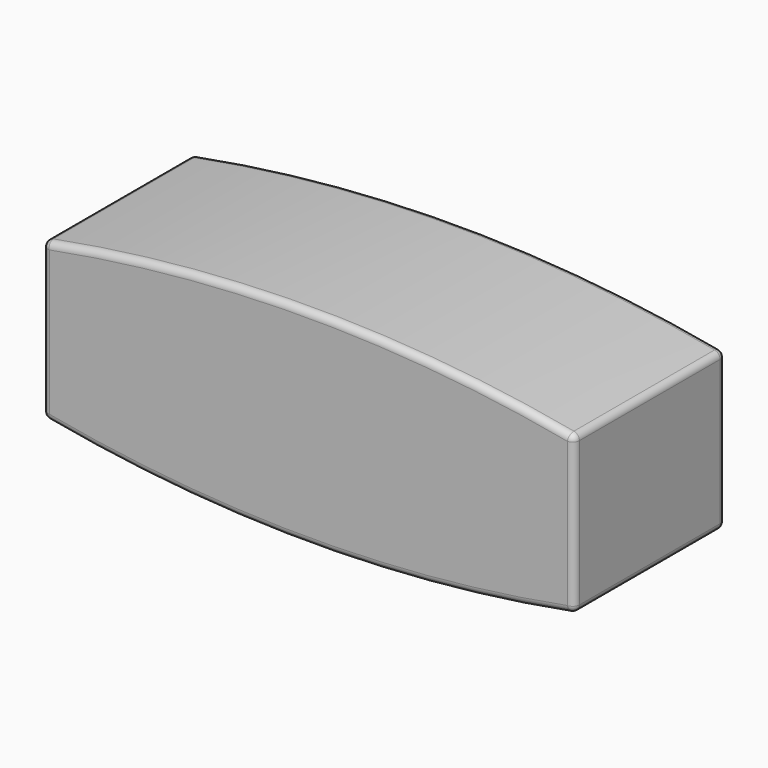
from build123d import *

# Parameters (mm, degrees)
F0_R     = 1.475
F1_DEPTH = 5
F0_R_2   = 2.5
F2_DEPTH = 2.6
F0_W     = 79.2
F0_H     = 28.2
F3_DEPTH = 23.2
F4_DEPTH = 11.6
F7_DEPTH = 28.2
F8_DEPTH = 28.2
F10_R    = 1


# Not quite as in the source:
# - two fillets or chamfers of one size are made in one step


with BuildPart() as f1:
    # F0 (on Top) → F1 (new body)
    with BuildSketch(Plane.XY):
        with Locations((-15, 8)):
            Circle(F0_R)
    extrude(amount=F1_DEPTH)


with BuildPart() as f1b:
    # F0 (on Top) → F1, piece 2 (new body)
    with BuildSketch(Plane.XY):
        with Locations((18.5, -8)):
            Circle(F0_R)
    extrude(amount=F1_DEPTH)


with BuildPart() as f2:
    # F0 (on Top) → F2 (new body)
    with BuildSketch(Plane.XY):
        with Locations((18.5, -8)):
            Circle(F0_R_2)
        with Locations((18.5, -8)):
            Circle(F0_R, mode=Mode.SUBTRACT)
    extrude(amount=F2_DEPTH)


with BuildPart() as f2b:
    # F0 (on Top) → F2, piece 2 (new body)
    with BuildSketch(Plane.XY):
        with Locations((-15, 8)):
            Circle(F0_R_2)
        with Locations((-15, 8)):
            Circle(F0_R, mode=Mode.SUBTRACT)
    extrude(amount=F2_DEPTH)


with BuildPart() as f3:
    # F0 (on Top) → F3 (new body)
    with BuildSketch(Plane.XY):
        Rectangle(F0_W, F0_H)
        Polygon((38, -10.5), (38, -12.5), (36, -12.5), (-36, -12.5), (-38, -12.5), (-38, -10.5), (-38, 10.5000000193), (-38, 12.5), (-36, 12.5), (36, 12.5), (38, 12.5), (38, 10.5), align=None, mode=Mode.SUBTRACT)
    extrude(amount=F3_DEPTH)

    # F5 (on face) → F7 (join, through all)
    with BuildSketch(Plane.XZ.offset(14.1)):
        with BuildLine():
            Line((-39.6, 23.2), (39.6, 23.2))
            ThreePointArc((39.6, 23.2), (0, 26.9675098342), (-39.6, 23.2))
        make_face()
    extrude(amount=-F7_DEPTH)

    # F6 (on face) → F8 (join, through all)
    with BuildSketch(Plane.XZ.offset(14.1)):
        with BuildLine():
            ThreePointArc((-39.6, 0), (0, -3.7675098342), (39.6, 0))
            Line((39.6, 0), (-39.6, 0))
        make_face()
    extrude(amount=-F8_DEPTH)

    # F10
    f10_edges = [f3.edges().sort_by_distance(p)[0] for p in [
        (-39.6, 14.1, 11.6),
        (-39.6, -14.1, 11.6),
        (39.6, 14.1, 11.6),
        (39.6, -14.1, 11.6),
        (39.6, 0, 0),
        (0, 14.1, -3.76751),
        (-39.6, 0, 0),
        (0, -14.1, -3.76751),
        (39.6, 0, 23.2),
        (0, -14.1, 26.96751),
        (0, 14.1, 26.96751),
        (-39.6, 0, 23.2),
    ]]
    fillet(f10_edges, radius=F10_R)


with BuildPart() as f4:
    # F0 (on Top) → F4 (new body)
    with BuildSketch(Plane.XY):
        with BuildLine():
            ThreePointArc((-36, 12.5), (-37.4142135555, 11.9142135692), (-38, 10.5000000193))
            ThreePointArc((-38, 10.5000000193), (-36.0000000097, 8.5), (-34, 10.5))
            ThreePointArc((-34, 10.5), (-34.5857864376, 11.9142135624), (-36, 12.5))
        make_face()
        with BuildLine():
            Line((-38, 12.5), (-38, 10.5000000193))
            ThreePointArc((-38, 10.5000000193), (-37.4142135555, 11.9142135692), (-36, 12.5))
            Line((-36, 12.5), (-38, 12.5))
        make_face()
    extrude(amount=F4_DEPTH)


with BuildPart() as f4b:
    # F0 (on Top) → F4, piece 2 (new body)
    with BuildSketch(Plane.XY):
        with BuildLine():
            ThreePointArc((-38, -10.5), (-37.4142135624, -11.9142135624), (-36, -12.5))
            ThreePointArc((-36, -12.5), (-34.5857864376, -11.9142135624), (-34, -10.5))
            ThreePointArc((-34, -10.5), (-36, -8.5), (-38, -10.5))
        make_face()
        with BuildLine():
            Line((-38, -12.5), (-36, -12.5))
            ThreePointArc((-36, -12.5), (-37.4142135624, -11.9142135624), (-38, -10.5))
            Line((-38, -10.5), (-38, -12.5))
        make_face()
    extrude(amount=F4_DEPTH)


with BuildPart() as f4c:
    # F0 (on Top) → F4, piece 3 (new body)
    with BuildSketch(Plane.XY):
        with BuildLine():
            ThreePointArc((36, 12.5), (34.5857864376, 9.0857864376), (38, 10.5))
            ThreePointArc((38, 10.5), (37.4142135624, 11.9142135624), (36, 12.5))
        make_face()
        with BuildLine():
            ThreePointArc((36, 12.5), (37.4142135624, 11.9142135624), (38, 10.5))
            Line((38, 10.5), (38, 12.5))
            Line((38, 12.5), (36, 12.5))
        make_face()
    extrude(amount=F4_DEPTH)


with BuildPart() as f4d:
    # F0 (on Top) → F4, piece 4 (new body)
    with BuildSketch(Plane.XY):
        with BuildLine():
            ThreePointArc((38, -10.5), (34.5857864376, -9.0857864376), (36, -12.5))
            ThreePointArc((36, -12.5), (37.4142135624, -11.9142135624), (38, -10.5))
        make_face()
        with BuildLine():
            Line((36, -12.5), (38, -12.5))
            Line((38, -12.5), (38, -10.5))
            ThreePointArc((38, -10.5), (37.4142135624, -11.9142135624), (36, -12.5))
        make_face()
    extrude(amount=F4_DEPTH)


solid = Compound([f1.part, f1b.part, f2.part, f2b.part, f3.part, f4.part, f4b.part, f4c.part, f4d.part])
